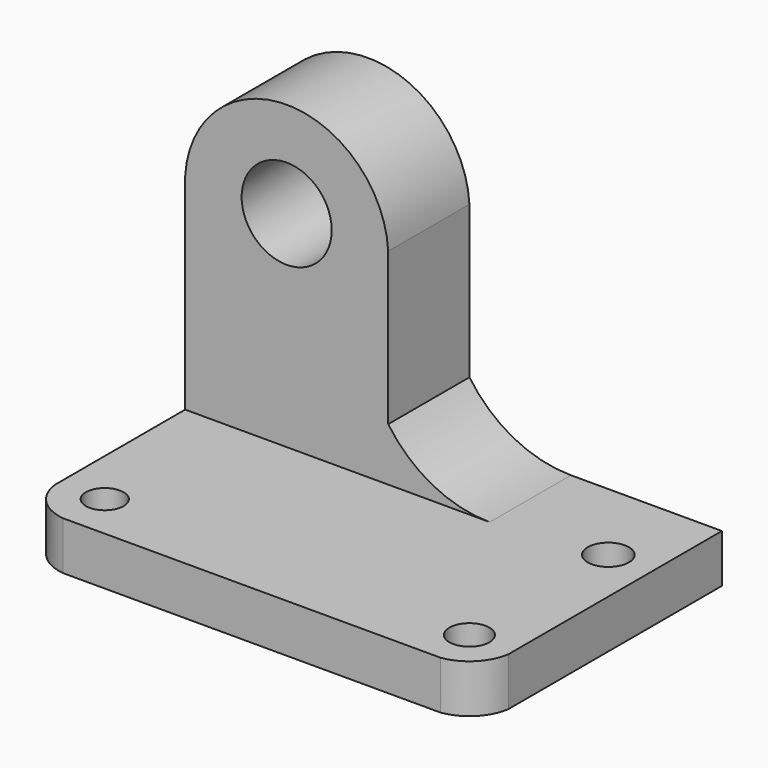
from build123d import *

# Parameters (mm, degrees)
F0_W     = 56.9855384529
F0_H     = 6.0439207591
F1_DEPTH = 38.1
F3_DEPTH = 12.7
F4_R     = 5.6337267147
F5_DEPTH = 25.4
F6_R     = 2.5763739366
F6_R_2   = 2.4951731212
F6_R_3   = 2.3565031445
F7_DEPTH = 25.4


with BuildPart() as f1:
    # F0 (on Front) → F1 (new body)
    with BuildSketch(Plane.XZ):
        with Locations((28.4927692264, 3.0219603796)):
            Rectangle(F0_W, F0_H)
    extrude(amount=F1_DEPTH)

    # F2 (on Front) → F3 (join)
    with BuildSketch(Plane.XZ):
        Polygon((0, 44.45), (0, 0), (38.1, 0), (38.1, 12.7), (25.4, 12.7), (25.4, 44.45), align=None)
    extrude(amount=F3_DEPTH)

    # F4 (on face) → F5 (cut)
    with BuildSketch(Plane.XZ.offset(12.7)):
        with BuildLine():
            ThreePointArc((0, 31.75), (12.7, 43.757902847), (25.4, 31.75))
            Line((25.4, 31.75), (25.4, 44.45))
            Line((25.4, 44.45), (0, 44.45))
            Line((0, 44.45), (0, 31.75))
        make_face()
        with Locations((12.7, 31.75)):
            Circle(F4_R)
        with BuildLine():
            Line((38.1, 12.7), (25.4, 12.7))
            ThreePointArc((25.4, 12.7), (30.9307359014, 7.8087797629), (38.1, 6.0439207591))
            Line((38.1, 6.0439207591), (38.1, 12.7))
        make_face()
    extrude(amount=-F5_DEPTH, mode=Mode.SUBTRACT)

    # F6 (on face) → F7 (cut)
    with BuildSketch(Plane.XY.offset(6.0439207591)):
        with BuildLine():
            ThreePointArc((56.9855384529, -33.4053455879), (55.411700833, -36.5261623801), (52.2908840407, -38.1))
            Line((52.2908840407, -38.1), (56.9855384529, -38.1))
            Line((56.9855384529, -38.1), (56.9855384529, -33.4053455879))
        make_face()
        with BuildLine():
            ThreePointArc((5.0487379712, -38.1), (1.6431313477, -36.4568686523), (0, -33.0512620288))
            Line((0, -33.0512620288), (0, -38.1))
            Line((0, -38.1), (5.0487379712, -38.1))
        make_face()
        with Locations((51.4632112468, -10.8606727939)):
            Circle(F6_R)
        with Locations((51.4632112468, -32.5776727939)):
            Circle(F6_R_2)
        with Locations((5.6993689856, -32.4006310144)):
            Circle(F6_R_3)
    extrude(amount=-F7_DEPTH, mode=Mode.SUBTRACT)


solid = f1.part
